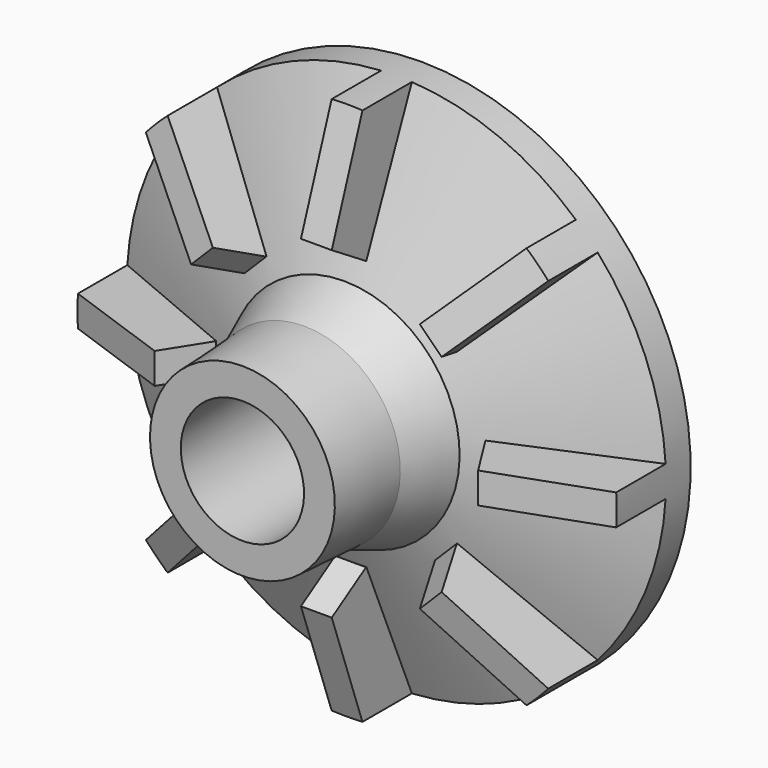
from build123d import *

# Parameters (mm, degrees)
F3_DEPTH        = 2
F3_COPIES_COUNT = 8
F4_W            = 13
F4_H            = 2


# Not quite as in the source:
# - a pattern or mirror of a feature is missing from the dataset's text; its kind, count and spacing are read off the source's solid


with BuildPart() as f1:
    # F0 (on Right) → F1 (revolve)
    with BuildSketch(Plane.YZ):
        Polygon((0, 12), (0, 8), (19.8, 8), (19.8, 15), (22.3, 15), (27.8, 32.7), (29, 32.7), (29, 35), (25, 35), (16.5, 15), (10, 12.5), align=None)
    revolve(axis=Axis((0, 14.5, 0), (0, 1, 0)))

    # F2 (on Right) → F3 (join, symmetric)
    with BuildSketch(Plane.YZ):
        Polygon((27, 35), (25, 35), (17, 35), (12, 21), (17.5625, 17.5), (19.5625, 17.5), align=None)
    f3 = extrude(amount=F3_DEPTH, both=True)

    # F3_copies: F3 ×8 about axis
    f3_copies_axis = Axis((0, 0, 0), (0, 1, 0))
    for i in range(1, F3_COPIES_COUNT):
        add(f3.rotate(f3_copies_axis, i * 360 / F3_COPIES_COUNT))

    # F4 (on Right) → F5 (revolve, cut)
    with BuildSketch(Plane.YZ):
        with Locations((22.5, 36)):
            Rectangle(F4_W, F4_H)
    revolve(axis=Axis((0, 14.5, 0), (0, 1, 0)), mode=Mode.SUBTRACT)


solid = f1.part
